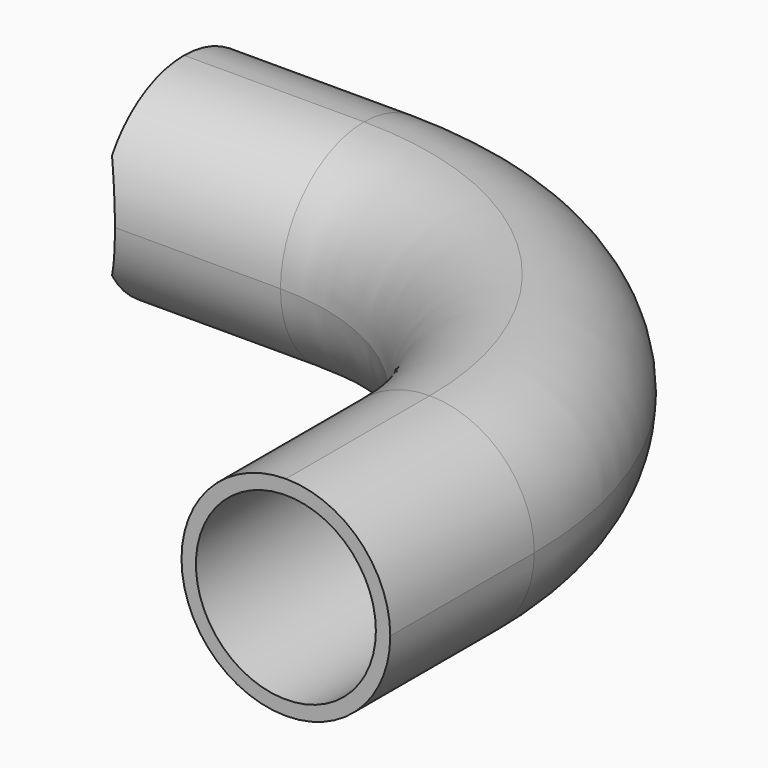
from build123d import *

# Parameters (mm, degrees)
F1_W     = 3.683
F1_H     = 3.683
F1_R     = 1.5875
F4_DEPTH = 3.683
F5_R     = 1.84149


# Not quite as in the source:
# - a fillet or chamfer is up to 0.001 mm smaller than in the source, because OpenCascade refuses the exact size


with BuildPart() as f2:
    # F2: sweep along a path in F0
    with BuildLine(Plane.XY) as f2_path:
        Line((0, 0), (0, 3.175))
        ThreePointArc((0, 3.175), (-1.7024337798, 7.2850387202), (-5.8124725, 8.9874725))
        Line((-5.8124725, 8.9874725), (-8.9874725, 8.9874725))
    # F1 (on Front) → F2 (sweep)
    with BuildSketch(Plane.XZ):
        Rectangle(F1_W, F1_H)
        Circle(F1_R, mode=Mode.SUBTRACT)
    sweep(path=f2_path.line)

    # F3 (on face) → F4 (cut, through all)
    with BuildSketch(Plane.XZ.offset(-7.1459725)):
        with BuildLine():
            Line((-8.9874725, 0), (-8.9874725, -0.933255592))
            ThreePointArc((-8.9874725, -0.933255592), (-8.7334725, 0), (-8.9874725, 0.933255592))
            Line((-8.9874725, 0.933255592), (-8.9874725, 0))
        make_face()
    extrude(amount=-F4_DEPTH, mode=Mode.SUBTRACT)

    # F5 (radius 1.8415 in the source; OpenCascade refuses exactly that, so slightly less here)
    f5_edges = [f2.edges().sort_by_distance(p)[0] for p in [
        (-3.004571, 5.982902, 1.8415),
        (-3.004571, 5.982902, -1.8415),
        (-0.400297, 8.587176, 1.8415),
        (-0.400297, 8.587176, -1.8415),
    ]]
    fillet(f5_edges, radius=F5_R)


solid = f2.part
